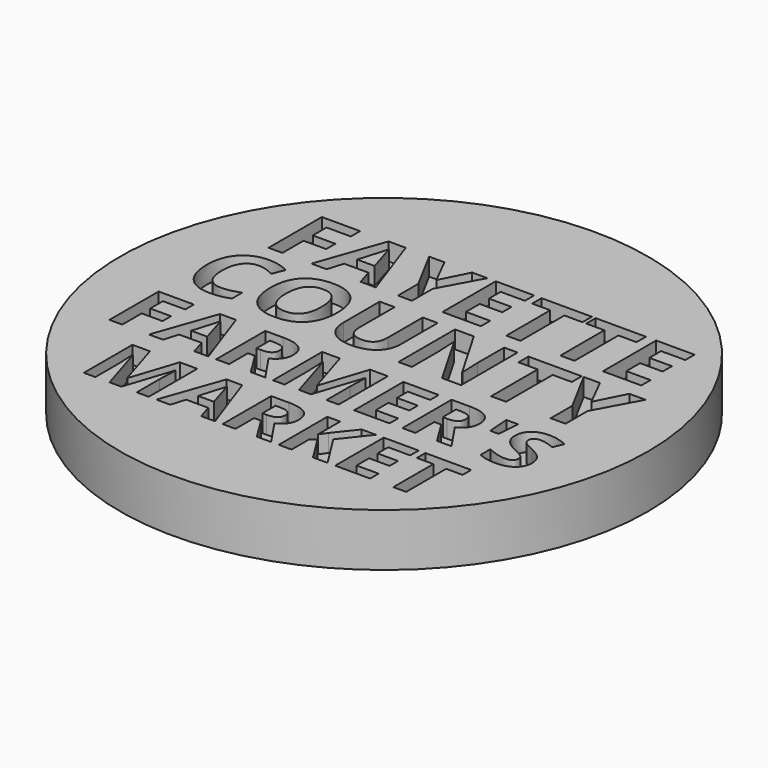
from build123d import *

# Parameters (mm, degrees)
F0_R           = 19.05
F1_DEPTH       = 3.81
F2_TEXT_SIZE   = 6.7376036172
F2_TEXT_SIZE_2 = 6.2150571893
F2_TEXT_SIZE_3 = 6.1338766886
F2_TEXT_SIZE_4 = 7.1381733021
F3_DEPTH       = 1.27


# Not quite as in the source:
# - Text() gives the source's letters only with a copy of the font that has no kerning and outlines rounded to 1/6400 em; it was checked with that copy


with BuildPart() as f1:
    # F0 (on Top) → F1 (new body)
    with BuildSketch(Plane.XY):
        Circle(F0_R)
    extrude(amount=F1_DEPTH)

    # F2 (on face) → F3 (cut)
    with BuildSketch(Plane.XY.offset(3.81)):
        with Locations((-13.7866547731, 6.053464493)):
            Text('FAYETTE', F2_TEXT_SIZE, font='Open Sans', font_style=FontStyle.BOLD, text_align=(TextAlign.LEFT, TextAlign.BOTTOM))
        with Locations((-15.2456378564, -6.4198332839)):
            Text("FARMER'S", F2_TEXT_SIZE_2, font='Open Sans', font_style=FontStyle.BOLD, text_align=(TextAlign.LEFT, TextAlign.BOTTOM))
        with Locations((-12.3270710295, -12.3643994853)):
            Text('MARKET', F2_TEXT_SIZE_3, font='Open Sans', font_style=FontStyle.BOLD, text_align=(TextAlign.LEFT, TextAlign.BOTTOM))
        with Locations((-15.0231588632, -0.2581388486)):
            Text('COUNTY', F2_TEXT_SIZE_4, font='Open Sans', font_style=FontStyle.BOLD, text_align=(TextAlign.LEFT, TextAlign.BOTTOM))
    extrude(amount=-F3_DEPTH, mode=Mode.SUBTRACT)


solid = f1.part
